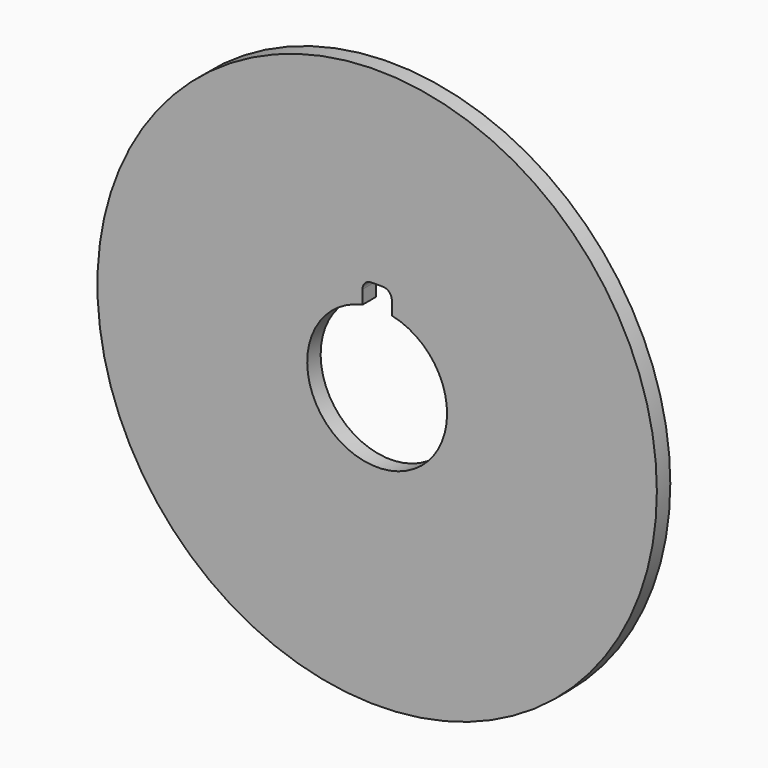
from build123d import *

# Parameters (mm, degrees)
F0_R     = 25.4
F0_R_2   = 6.35
F1_DEPTH = 1.524
F2_W     = 2.667
F2_H     = 8.255
F3_DEPTH = 73
F4_R     = 0.8128


# Not quite as in the source:
# - an extrude ends at something that could not be found from the text; its depth is read off the source's solid


with BuildPart() as f1:
    # F0 (on Front) → F1 (new body)
    with BuildSketch(Plane.XZ):
        Circle(F0_R)
        Circle(F0_R_2, mode=Mode.SUBTRACT)
    extrude(amount=F1_DEPTH)

    # F2 (on Front) → F3 (cut, through all)
    with BuildSketch(Plane.XZ):
        with Locations((0, 4.1275)):
            Rectangle(F2_W, F2_H)
    extrude(amount=F3_DEPTH, mode=Mode.SUBTRACT)

    # F4
    f4_edges = [f1.edges().sort_by_distance(p)[0] for p in [
        (-1.3335, -0.762, 8.255),
        (1.3335, -0.762, 8.255),
    ]]
    fillet(f4_edges, radius=F4_R)


solid = f1.part
